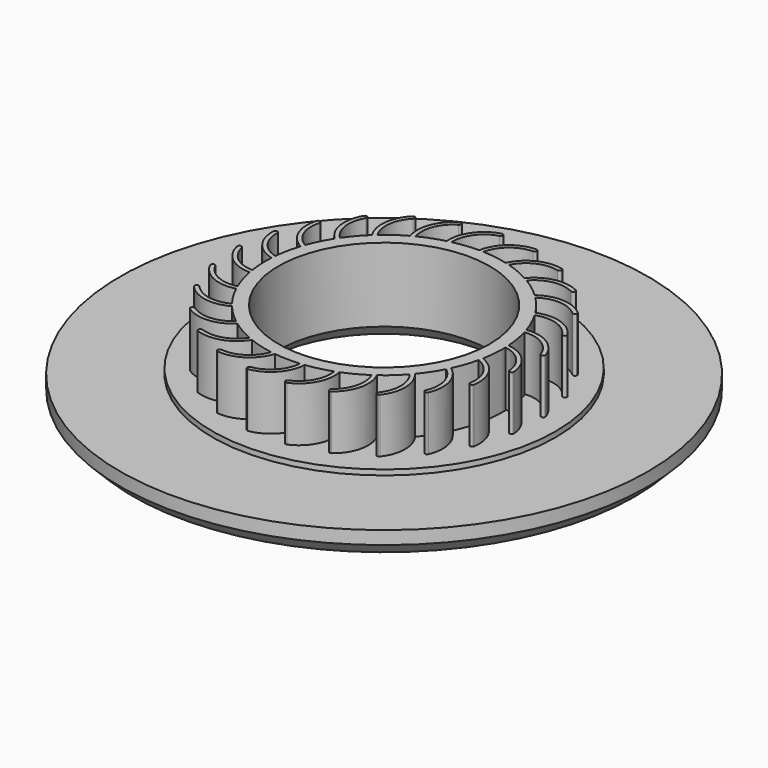
from build123d import *
from build123d import SkipClean  # not in build123d's __all__

# Parameters (mm, degrees)
F0_R     = 50
F1_DEPTH = 5
F2_R     = 32.5
F3_DEPTH = 1
F4_SIZE  = 2.5
F6_DEPTH = 10.5
F7_DEPTH = 0.2
F8_R     = 20
F9_DEPTH = 16.501
F10_SIZE = 2.5


# Not quite as in the source:
# - after a boolean that leaves OpenCascade's solid faulty, fix() repairs it


with BuildPart() as f1:
    # F0 (on Top) → F1 (new body)
    with BuildSketch(Plane.XY):
        Circle(F0_R)
    extrude(amount=F1_DEPTH)

    # F2 (on face) → F3 (join)
    with BuildSketch(Plane.XY.offset(5)):
        Circle(F2_R)
    extrude(amount=F3_DEPTH)

    # F4
    f4_edges = [f1.edges().sort_by_distance(p)[0] for p in [
        (-50, 0, 0),
    ]]
    chamfer(f4_edges, length=F4_SIZE)

    # F5 (on face) → F6 (join)
    with BuildSketch(Plane.XY.offset(6)):
        with BuildLine():
            ThreePointArc((22.4919640181, 0.601294112), (22.4774451189, 1.0072045119), (22.4556013896, 1.4127866894))
            ThreePointArc((22.4556013896, 1.4127866894), (22.1739675521, 3.8164332825), (21.6358018438, 6.1759273455))
            ThreePointArc((21.6358018438, 6.1759273455), (21.5207932709, 6.5654746204), (21.3987716166, 6.9528823734))
            ThreePointArc((21.3987716166, 6.9528823734), (20.528223224, 9.2109745015), (19.4201826687, 11.3625043505))
            ThreePointArc((19.4201826687, 11.3625043505), (19.2119108338, 11.7112118124), (18.9973783238, 12.056102887))
            ThreePointArc((18.9973783238, 12.056102887), (17.5926151331, 14.026756317), (15.9843219941, 15.8351334187))
            ThreePointArc((15.9843219941, 15.8351334187), (15.6958733825, 16.1210904954), (15.4023098834, 16.401794117))
            ThreePointArc((15.4023098834, 16.401794117), (13.5515983324, 17.9611854463), (11.5441075824, 19.3127828167))
            ThreePointArc((11.5441075824, 19.3127828167), (11.1936064813, 19.5180217733), (10.8394576673, 19.716900301))
            ThreePointArc((10.8394576673, 19.716900301), (8.6590847692, 20.7670472374), (6.3785344351, 21.5769390429))
            ThreePointArc((6.3785344351, 21.5769390429), (5.9880041176, 21.6885639609), (5.5955224612, 21.7931211254))
            ThreePointArc((5.5955224612, 21.7931211254), (3.222489064, 22.2680390747), (0.8121745106, 22.4853368346))
            ThreePointArc((0.8121745106, 22.4853368346), (0.4061534328, 22.49633391), (0, 22.5))
            ThreePointArc((0, 22.5), (-2.4165874806, 22.3698481208), (-4.8052173254, 21.9808982177))
            ThreePointArc((-4.8052173254, 21.9808982177), (-5.2012173658, 21.8905764637), (-5.5955224612, 21.7931211254))
            ThreePointArc((-5.5955224612, 21.7931211254), (-7.9038209461, 21.066077339), (-10.1206796845, 20.0953189256))
            ThreePointArc((-10.1206796845, 20.0953189256), (-10.4817765486, 19.9093535903), (-10.8394576673, 19.716900301))
            ThreePointArc((-10.8394576673, 19.716900301), (-12.8944282734, 18.4386474423), (-14.8002225178, 16.9470768401))
            ThreePointArc((-14.8002225178, 16.9470768401), (-15.1037271616, 16.6771528094), (-15.4023098834, 16.401794117))
            ThreePointArc((-15.4023098834, 16.401794117), (-17.0748312499, 14.6526495142), (-18.5498129388, 12.7339875897))
            ThreePointArc((-18.5498129388, 12.7339875897), (-18.7766550494, 12.3970651831), (-18.9973783238, 12.056102887))
            ThreePointArc((-18.9973783238, 12.056102887), (-20.1823597822, 9.9459717285), (-21.1338503915, 7.7207750668))
            ThreePointArc((-21.1338503915, 7.7207750668), (-21.2697766448, 7.3380243582), (-21.3987716166, 6.9528823734))
            ThreePointArc((-21.3987716166, 6.9528823734), (-22.0217564237, 4.6143519603), (-22.3899702992, 2.2224378513))
            ThreePointArc((-22.3899702992, 2.2224378513), (-22.4264399487, 1.8179084755), (-22.4556013896, 1.4127866894))
            ThreePointArc((-22.4556013896, 1.4127866894), (-22.4774451189, -1.0072045119), (-22.2392460284, -3.4155433079))
            ThreePointArc((-22.2392460284, -3.4155433079), (-22.1739675521, -3.8164332825), (-22.1014631414, -4.2160795782))
            ThreePointArc((-22.1014631414, -4.2160795782), (-21.5207932709, -6.5654746204), (-20.6911481395, -8.8389133196))
            ThreePointArc((-20.6911481395, -8.8389133196), (-20.528223224, -9.2109745015), (-20.3586086805, -9.5800340602))
            ThreePointArc((-20.3586086805, -9.5800340602), (-19.2119108338, -11.7112118124), (-17.8429493162, -13.7069019001))
            ThreePointArc((-17.8429493162, -13.7069019001), (-17.5926151331, -14.026756317), (-17.3365479625, -14.3420397693))
            ThreePointArc((-17.3365479625, -14.3420397693), (-15.6958733825, -16.1210904954), (-13.8736123656, -17.7136354238))
            ThreePointArc((-13.8736123656, -17.7136354238), (-13.5515983324, -17.9611854463), (-13.2251681766, -18.2028823734))
            ThreePointArc((-13.2251681766, -18.2028823734), (-11.1936064813, -19.5180217733), (-9.0325453265, -20.6073560877))
            ThreePointArc((-9.0325453265, -20.6073560877), (-8.6590847692, -20.7670472374), (-8.2828024354, -20.9199709325))
            ThreePointArc((-8.2828024354, -20.9199709325), (-5.9880041176, -21.6885639609), (-3.6239302452, -22.20624078))
            ThreePointArc((-3.6239302452, -22.20624078), (-3.222489064, -22.2680390747), (-2.8199977552, -22.3225807796))
            ThreePointArc((-2.8199977552, -22.3225807796), (-0.4061534328, -22.49633391), (2.0123897013, -22.4098256952))
            ThreePointArc((2.0123897013, -22.4098256952), (2.4165874806, -22.3698481208), (2.8199977552, -22.3225807796))
            ThreePointArc((2.8199977552, -22.3225807796), (5.2012173658, -21.8905764637), (7.5222638018, -21.2053188445))
            ThreePointArc((7.5222638018, -21.2053188445), (7.9038209461, -21.066077339), (8.2828024354, -20.9199709325))
            ThreePointArc((8.2828024354, -20.9199709325), (10.4817765486, -19.9093535903), (12.5594864028, -18.668403823))
            ThreePointArc((12.5594864028, -18.668403823), (12.8944282734, -18.4386474423), (13.2251681766, -18.2028823734))
            ThreePointArc((13.2251681766, -18.2028823734), (15.1037271616, -16.6771528094), (16.8075502824, -14.9584843318))
            ThreePointArc((16.8075502824, -14.9584843318), (17.0748312499, -14.6526495142), (17.3365479625, -14.3420397693))
            ThreePointArc((17.3365479625, -14.3420397693), (18.7766550494, -12.3970651831), (19.999533964, -10.3086682565))
            ThreePointArc((19.999533964, -10.3086682565), (20.1823597822, -9.9459717285), (20.3586086805, -9.5800340602))
            ThreePointArc((20.3586086805, -9.5800340602), (21.2697766448, -7.3380243582), (21.9348733735, -5.011120642))
            ThreePointArc((21.9348733735, -5.011120642), (22.0217564237, -4.6143519603), (22.1014631414, -4.2160795782))
            ThreePointArc((22.1014631414, -4.2160795782), (22.4001442036, -2.1174370497), (22.5, 0))
            ThreePointArc((22.5, 0), (22.4979909148, 0.300673904), (22.4919640181, 0.601294112))
        make_face()
        with BuildLine():
            ThreePointArc((-13.9116834444, 24.2717188462), (-13.846454671, 24.7564653989), (-14.2990440405, 24.9419293466))
            ThreePointArc((-14.2990440405, 24.9419293466), (-14.386541076, 24.8915635481), (-14.4738607094, 24.8408908086))
            ThreePointArc((-14.4738607094, 24.8408908086), (-16.4354533618, 20.7860793054), (-15.4023098834, 16.401794117))
            ThreePointArc((-15.4023098834, 16.401794117), (-15.1037271616, 16.6771528094), (-14.8002225178, 16.9470768401))
            ThreePointArc((-14.8002225178, 16.9470768401), (-15.6326549951, 20.7642722553), (-13.9116834444, 24.2717188462))
        make_face()
        with BuildLine():
            ThreePointArc((-7.438491306, 26.9688731522), (-7.254760249, 27.4221687642), (-7.647007683, 27.7143604201))
            ThreePointArc((-7.647007683, 27.7143604201), (-7.744281303, 27.6873365837), (-7.8414594274, 27.6599713313))
            ThreePointArc((-7.8414594274, 27.6599713313), (-10.7498156547, 24.2203774431), (-10.8394576673, 19.716900301))
            ThreePointArc((-10.8394576673, 19.716900301), (-10.4817765486, 19.9093535903), (-10.1206796845, 20.0953189256))
            ThreePointArc((-10.1206796845, 20.0953189256), (-9.9776618678, 23.9996076664), (-7.438491306, 26.9688731522))
        make_face()
        with BuildLine():
            ThreePointArc((-0.4979114021, 27.9714739734), (-0.2072225594, 28.3648364144), (-0.514481709, 28.7453963022))
            ThreePointArc((-0.514481709, 28.7453963022), (-0.6154198542, 28.7434124349), (-0.7163504107, 28.741074129))
            ThreePointArc((-0.7163504107, 28.741074129), (-4.3887274949, 26.1328201898), (-5.5955224612, 21.7931211254))
            ThreePointArc((-5.5955224612, 21.7931211254), (-5.2012173658, 21.8905764637), (-4.8052173254, 21.9808982177))
            ThreePointArc((-4.8052173254, 21.9808982177), (-3.69573555, 25.7269594634), (-0.4979114021, 27.9714739734))
        make_face()
        with BuildLine():
            ThreePointArc((6.4739541065, 27.216524213), (6.8533356857, 27.5252370741), (6.6503710429, 27.9702532165))
            ThreePointArc((6.6503710429, 27.9702532165), (6.5521106873, 27.9934339719), (6.4537695369, 28.0162695369))
            ThreePointArc((6.4537695369, 28.0162695369), (2.2481205539, 26.4032417342), (0, 22.5))
            ThreePointArc((0, 22.5), (0.4061534328, 22.49633391), (0.8121745106, 22.4853368346))
            ThreePointArc((0.8121745106, 22.4853368346), (2.8184074243, 25.8377917802), (6.4739541065, 27.216524213))
        make_face()
        with BuildLine():
            ThreePointArc((13.039037269, 24.7514601409), (13.4832736448, 24.9561258576), (13.3973565237, 25.4376362537))
            ThreePointArc((13.3973565237, 25.4376362537), (13.3079480174, 25.4845250999), (13.2183754092, 25.5310996932))
            ThreePointArc((13.2183754092, 25.5310996932), (8.7437109204, 25.014650496), (5.5955224612, 21.7931211254))
            ThreePointArc((5.5955224612, 21.7931211254), (5.9880041176, 21.6885639609), (6.3785344351, 21.5769390429))
            ThreePointArc((6.3785344351, 21.5769390429), (9.1554594948, 24.3251406147), (13.039037269, 24.7514601409))
        make_face()
        with BuildLine():
            ThreePointArc((18.7848297657, 20.7311707986), (19.2660079329, 20.8189294714), (19.3025368222, 21.3066790521))
            ThreePointArc((19.3025368222, 21.3066790521), (19.2275980304, 21.3743297902), (19.1524221407, 21.4417169589))
            ThreePointArc((19.1524221407, 21.4417169589), (14.6899017726, 22.0542967698), (10.8394576673, 19.716900301))
            ThreePointArc((10.8394576673, 19.716900301), (11.1936064813, 19.5180217733), (11.5441075824, 19.3127828167))
            ThreePointArc((11.5441075824, 19.3127828167), (14.9172403738, 21.2840514028), (18.7848297657, 20.7311707986))
        make_face()
        with BuildLine():
            ThreePointArc((23.3503023224, 15.4082657512), (23.8381880871, 15.3736031798), (23.9948677424, 15.8369448451))
            ThreePointArc((23.9948677424, 15.8369448451), (23.9391073449, 15.9211067306), (23.8830517514, 16.005072291))
            ThreePointArc((23.8830517514, 16.005072291), (19.7130720707, 17.7081904675), (15.4023098834, 16.401794117))
            ThreePointArc((15.4023098834, 16.401794117), (15.6958733825, 16.1210904954), (15.9843219941, 15.8351334187))
            ThreePointArc((15.9843219941, 15.8351334187), (19.7417161784, 16.905606964), (23.3503023224, 15.4082657512))
        make_face()
        with BuildLine():
            ThreePointArc((26.4485895078, 9.117202699), (26.9125272131, 8.9622968602), (27.1795128753, 9.3721171493))
            ThreePointArc((27.1795128753, 9.3721171493), (27.1464345031, 9.4675019813), (27.1130213849, 9.5627700685))
            ThreePointArc((27.1130213849, 9.5627700685), (23.4975975511, 12.2494134319), (18.9973783238, 12.056102887))
            ThreePointArc((18.9973783238, 12.056102887), (19.2119108338, 11.7112118124), (19.4201826687, 11.3625043505))
            ThreePointArc((19.4201826687, 11.3625043505), (23.3257473505, 11.4649210651), (26.4485895078, 9.117202699))
        make_face()
        with BuildLine():
            ThreePointArc((27.8850145434, 2.2532722704), (28.2958532769, 1.9878564679), (28.6563692551, 2.3184048648))
            ThreePointArc((28.6563692551, 2.3184048648), (28.6480513439, 2.4190192636), (28.63938017, 2.5196038332))
            ThreePointArc((28.63938017, 2.5196038332), (25.8056825592, 6.0209607002), (21.3987716166, 6.9528823734))
            ThreePointArc((21.3987716166, 6.9528823734), (21.5207932709, 6.5654746204), (21.6358018438, 6.1759273455))
            ThreePointArc((21.6358018438, 6.1759273455), (25.4441360304, 5.3038520107), (27.8850145434, 2.2532722704))
        make_face()
        with BuildLine():
            ThreePointArc((28.3326405638, -4.8809813239), (28.3496057586, -4.7814593311), (28.3662213708, -4.6818783775))
            ThreePointArc((28.3662213708, -4.6818783775), (26.4923016254, -0.5858111358), (22.4556013896, 1.4127866894))
            ThreePointArc((22.4556013896, 1.4127866894), (22.4774451189, 1.0072045119), (22.4919640181, 0.601294112))
            ThreePointArc((22.4919640181, 0.601294112), (25.9637760666, -1.1904775717), (27.5693215612, -4.7522395418))
            ThreePointArc((27.5693215612, -4.7522395418), (27.9012468145, -5.1114882571), (28.3326405638, -4.8809813239))
        make_face()
        with BuildLine():
            ThreePointArc((26.2286678657, -11.773677505), (26.2698501808, -11.681501251), (26.3107085592, -11.5891809509))
            ThreePointArc((26.3107085592, -11.5891809509), (25.5143119486, -7.1557743037), (22.1014631414, -4.2160795782))
            ThreePointArc((22.1014631414, -4.2160795782), (22.0217564237, -4.6143519603), (21.9348733735, -5.011120642))
            ThreePointArc((21.9348733735, -5.011120642), (24.8520165645, -7.61000507), (25.5213467125, -11.4591506661))
            ThreePointArc((25.5213467125, -11.4591506661), (25.7535024011, -11.8896593762), (26.2286678657, -11.773677505))
        make_face()
        with BuildLine():
            ThreePointArc((22.4766515033, -17.9265902279), (22.5394633025, -17.8475514857), (22.6019971648, -17.7682926631))
            ThreePointArc((22.6019971648, -17.7682926631), (22.9331642171, -13.276113855), (20.3586086805, -9.5800340602))
            ThreePointArc((20.3586086805, -9.5800340602), (20.1823597822, -9.9459717285), (19.999533964, -10.3086682565))
            ThreePointArc((19.999533964, -10.3086682565), (22.1787134623, -13.5513679622), (21.8697717889, -17.4460412103))
            ThreePointArc((21.8697717889, -17.4460412103), (21.9875707171, -17.9207594696), (22.4766515033, -17.9265902279))
        make_face()
        with BuildLine():
            ThreePointArc((17.3123444636, -22.9531093574), (17.3928390506, -22.8921744219), (17.4731191642, -22.8309572001))
            ThreePointArc((17.4731191642, -22.8309572001), (18.9110414355, -18.5622663467), (17.3365479625, -14.3420397693))
            ThreePointArc((17.3365479625, -14.3420397693), (17.0748312499, -14.6526495142), (16.8075502824, -14.9584843318))
            ThreePointArc((16.8075502824, -14.9584843318), (18.1118402256, -18.6412485668), (16.8440386724, -22.3367328231))
            ThreePointArc((16.8440386724, -22.3367328231), (16.8400791003, -22.8258323375), (17.3123444636, -22.9531093574))
        make_face()
        with BuildLine():
            ThreePointArc((11.0602391509, -26.5374002103), (11.1533587547, -26.4983978476), (11.2463408249, -26.4590687298))
            ThreePointArc((11.2463408249, -26.4590687298), (13.7006683705, -22.6820833765), (13.2251681766, -18.2028823734))
            ThreePointArc((13.2251681766, -18.2028823734), (12.8944282734, -18.4386474423), (12.5594864028, -18.668403823))
            ThreePointArc((12.5594864028, -18.668403823), (12.9069334569, -22.5598309663), (10.7599326581, -25.8239253639))
            ThreePointArc((10.7599326581, -25.8239253639), (10.6344633801, -26.2966742122), (11.0602391509, -26.5374002103))
        make_face()
        with BuildLine():
            ThreePointArc((4.1131783357, -28.4542486103), (4.213071909, -28.4396294823), (4.3129135304, -28.4246596616))
            ThreePointArc((4.3129135304, -28.4246596616), (7.6294319243, -25.376701689), (8.2828024354, -20.9199709325))
            ThreePointArc((8.2828024354, -20.9199709325), (7.9038209461, -21.066077339), (7.5222638018, -21.2053188445))
            ThreePointArc((7.5222638018, -21.2053188445), (6.8910365907, -25.0608962169), (3.9997405026, -27.6885057004))
            ThreePointArc((3.9997405026, -27.6885057004), (3.760645215, -28.1151993337), (4.1131783357, -28.4542486103))
        make_face()
        with BuildLine():
            ThreePointArc((-3.0923286016, -28.5832119227), (-2.9919377393, -28.5938946029), (-2.891509983, -28.6042246883))
            ThreePointArc((-2.891509983, -28.6042246883), (1.0788102112, -26.4768085053), (2.8199977552, -22.3225807796))
            ThreePointArc((2.8199977552, -22.3225807796), (2.4165874806, -22.3698481208), (2.0123897013, -22.4098256952))
            ThreePointArc((2.0123897013, -22.4098256952), (0.442150552, -25.9872931907), (-3.0117700587, -27.8133153925))
            ThreePointArc((-3.0117700587, -27.8133153925), (-3.3494681197, -28.1671430805), (-3.0923286016, -28.5832119227))
        make_face()
        with BuildLine():
            ThreePointArc((-10.10353316, -26.9161869083), (-10.0089529358, -26.9515001647), (-9.9142492899, -26.9864810788))
            ThreePointArc((-9.9142492899, -26.9864810788), (-5.539597115, -25.9132800684), (-2.8199977552, -22.3225807796))
            ThreePointArc((-2.8199977552, -22.3225807796), (-3.222489064, -22.2680390747), (-3.6239302452, -22.20624078))
            ThreePointArc((-3.6239302452, -22.20624078), (-6.0345174319, -25.2808129587), (-9.8340400307, -26.1905121883))
            ThreePointArc((-9.8340400307, -26.1905121883), (-10.2491220539, -26.4492416362), (-10.10353316, -26.9161869083))
        make_face()
        with BuildLine():
            ThreePointArc((-16.4798955719, -23.5579188797), (-16.397068809, -23.6156438505), (-16.3140398519, -23.6730776138))
            ThreePointArc((-16.3140398519, -23.6730776138), (-11.8099311813, -23.7215249424), (-8.2828024354, -20.9199709325))
            ThreePointArc((-8.2828024354, -20.9199709325), (-8.6590847692, -20.7670472374), (-9.0325453265, -20.6073560877))
            ThreePointArc((-9.0325453265, -20.6073560877), (-12.1320144922, -22.9858462722), (-16.0384011005, -22.9220627813))
            ThreePointArc((-16.0384011005, -22.9220627813), (-16.5047859559, -23.0694370663), (-16.4798955719, -23.5579188797))
        make_face()
        with BuildLine():
            ThreePointArc((-21.8207655361, -18.7194201678), (-21.7548965448, -18.7959297808), (-21.6887592912, -18.8722076189))
            ThreePointArc((-21.6887592912, -18.8722076189), (-17.3382038376, -20.0392591626), (-13.2251681766, -18.2028823734))
            ThreePointArc((-13.2251681766, -18.2028823734), (-13.5515983324, -17.9611854463), (-13.8736123656, -17.7136354238))
            ThreePointArc((-13.8736123656, -17.7136354238), (-17.4672124636, -19.2465943284), (-21.235010444, -18.2133358683))
            ThreePointArc((-21.235010444, -18.2133358683), (-21.7233934559, -18.2400949221), (-21.8207655361, -18.7194201678))
        make_face()
        with BuildLine():
            ThreePointArc((-25.7905565505, -12.7047114416), (-25.7457841217, -12.7951983164), (-25.7006942185, -12.8855274121))
            ThreePointArc((-25.7006942185, -12.8855274121), (-21.7770533813, -15.0978530303), (-17.3365479625, -14.3420397693))
            ThreePointArc((-17.3365479625, -14.3420397693), (-17.5926151331, -14.026756317), (-17.8429493162, -13.7069019001))
            ThreePointArc((-17.8429493162, -13.7069019001), (-21.7048812359, -14.2980080789), (-25.0973459844, -12.3601980787))
            ThreePointArc((-25.0973459844, -12.3601980787), (-25.577040252, -12.2646605315), (-25.7905565505, -12.7047114416))
        make_face()
        with BuildLine():
            ThreePointArc((-28.1398320458, -5.8917189709), (-28.1189693959, -5.9904974844), (-28.0977600075, -6.0892021283))
            ThreePointArc((-28.0977600075, -6.0892021283), (-24.8475705707, -9.2077932662), (-20.3586086805, -9.5800340602))
            ThreePointArc((-20.3586086805, -9.5800340602), (-20.528223224, -9.2109745015), (-20.6911481395, -8.8389133196))
            ThreePointArc((-20.6911481395, -8.8389133196), (-24.5787524952, -8.4510253974), (-27.3827229751, -5.7304235863))
            ThreePointArc((-27.3827229751, -5.7304235863), (-27.8235875433, -5.5185924135), (-28.1398320458, -5.8917189709))
        make_face()
        with BuildLine():
            ThreePointArc((-28.7209784027, 1.291471871), (-28.7253364086, 1.1906083361), (-28.7293401989, 1.0897301196))
            ThreePointArc((-28.7293401989, 1.0897301196), (-26.3568235181, -2.7391739872), (-22.1014631414, -4.2160795782))
            ThreePointArc((-22.1014631414, -4.2160795782), (-22.1739675521, -3.8164332825), (-22.2392460284, -3.4155433079))
            ThreePointArc((-22.2392460284, -3.4155433079), (-25.9082503409, -2.0730337095), (-27.9475427746, 1.2594144951))
            ThreePointArc((-27.9475427746, 1.2594144951), (-28.3218765012, 1.5742291618), (-28.7209784027, 1.291471871))
        make_face()
        with BuildLine():
            ThreePointArc((-26.7563156777, 8.170118932), (-27.040597798, 8.5681361292), (-27.4974800581, 8.3935147856))
            ThreePointArc((-27.4974800581, 8.3935147856), (-27.5267848904, 8.2969038561), (-27.5557502865, 8.2001906164))
            ThreePointArc((-27.5557502865, 8.2001906164), (-26.2099803103, 3.9015576673), (-22.4556013896, 1.4127866894))
            ThreePointArc((-22.4556013896, 1.4127866894), (-22.4264399487, 1.8179084755), (-22.3899702992, 2.2224378513))
            ThreePointArc((-22.3899702992, 2.2224378513), (-25.6098375338, 4.4352143104), (-26.7563156777, 8.170118932))
        make_face()
        with BuildLine():
            ThreePointArc((-23.8838908639, 14.5674647488), (-24.0602588868, 15.0236755923), (-24.5462139128, 14.9681622969))
            ThreePointArc((-24.5462139128, 14.9681622969), (-24.5986242411, 14.8818743929), (-24.6507312407, 14.7954029786))
            ThreePointArc((-24.6507312407, 14.7954029786), (-24.416267646, 10.2971401047), (-21.3987716166, 6.9528823734))
            ThreePointArc((-21.3987716166, 6.9528823734), (-21.2697766448, 7.3380243582), (-21.1338503915, 7.7207750668))
            ThreePointArc((-21.1338503915, 7.7207750668), (-23.7022644481, 10.6647815037), (-23.8838908639, 14.5674647488))
        make_face()
        with BuildLine():
            ThreePointArc((-19.5107533484, 20.0494831801), (-19.5681254223, 20.5352222647), (-20.0526188727, 20.6023051222))
            ThreePointArc((-20.0526188727, 20.6023051222), (-20.1248415633, 20.5317620299), (-20.1968160919, 20.460965758))
            ThreePointArc((-20.1968160919, 20.460965758), (-21.0883910888, 16.0457153591), (-18.9973783238, 12.056102887))
            ThreePointArc((-18.9973783238, 12.056102887), (-18.7766550494, 12.3970651831), (-18.5498129388, 12.7339875897))
            ThreePointArc((-18.5498129388, 12.7339875897), (-20.3053909162, 16.2242412527), (-19.5107533484, 20.0494831801))
        make_face()
    extrude(amount=F6_DEPTH)

    # F5 (on face) → F7 (cut)
    with BuildSketch(Plane.XY.offset(6)):
        with BuildLine():
            ThreePointArc((-10.10353316, -26.9161869083), (-10.0089529358, -26.9515001647), (-9.9142492899, -26.9864810788))
            ThreePointArc((-9.9142492899, -26.9864810788), (-5.539597115, -25.9132800684), (-2.8199977552, -22.3225807796))
            ThreePointArc((-2.8199977552, -22.3225807796), (-3.222489064, -22.2680390747), (-3.6239302452, -22.20624078))
            ThreePointArc((-3.6239302452, -22.20624078), (-6.0345174319, -25.2808129587), (-9.8340400307, -26.1905121883))
            ThreePointArc((-9.8340400307, -26.1905121883), (-10.2491220539, -26.4492416362), (-10.10353316, -26.9161869083))
        make_face()
        with BuildLine():
            ThreePointArc((-16.4798955719, -23.5579188797), (-16.397068809, -23.6156438505), (-16.3140398519, -23.6730776138))
            ThreePointArc((-16.3140398519, -23.6730776138), (-11.8099311813, -23.7215249424), (-8.2828024354, -20.9199709325))
            ThreePointArc((-8.2828024354, -20.9199709325), (-8.6590847692, -20.7670472374), (-9.0325453265, -20.6073560877))
            ThreePointArc((-9.0325453265, -20.6073560877), (-12.1320144922, -22.9858462722), (-16.0384011005, -22.9220627813))
            ThreePointArc((-16.0384011005, -22.9220627813), (-16.5047859559, -23.0694370663), (-16.4798955719, -23.5579188797))
        make_face()
        with BuildLine():
            ThreePointArc((-21.8207655361, -18.7194201678), (-21.7548965448, -18.7959297808), (-21.6887592912, -18.8722076189))
            ThreePointArc((-21.6887592912, -18.8722076189), (-17.3382038376, -20.0392591626), (-13.2251681766, -18.2028823734))
            ThreePointArc((-13.2251681766, -18.2028823734), (-13.5515983324, -17.9611854463), (-13.8736123656, -17.7136354238))
            ThreePointArc((-13.8736123656, -17.7136354238), (-17.4672124636, -19.2465943284), (-21.235010444, -18.2133358683))
            ThreePointArc((-21.235010444, -18.2133358683), (-21.7233934559, -18.2400949221), (-21.8207655361, -18.7194201678))
        make_face()
        with BuildLine():
            ThreePointArc((-25.7905565505, -12.7047114416), (-25.7457841217, -12.7951983164), (-25.7006942185, -12.8855274121))
            ThreePointArc((-25.7006942185, -12.8855274121), (-21.7770533813, -15.0978530303), (-17.3365479625, -14.3420397693))
            ThreePointArc((-17.3365479625, -14.3420397693), (-17.5926151331, -14.026756317), (-17.8429493162, -13.7069019001))
            ThreePointArc((-17.8429493162, -13.7069019001), (-21.7048812359, -14.2980080789), (-25.0973459844, -12.3601980787))
            ThreePointArc((-25.0973459844, -12.3601980787), (-25.577040252, -12.2646605315), (-25.7905565505, -12.7047114416))
        make_face()
        with BuildLine():
            ThreePointArc((-28.1398320458, -5.8917189709), (-28.1189693959, -5.9904974844), (-28.0977600075, -6.0892021283))
            ThreePointArc((-28.0977600075, -6.0892021283), (-24.8475705707, -9.2077932662), (-20.3586086805, -9.5800340602))
            ThreePointArc((-20.3586086805, -9.5800340602), (-20.528223224, -9.2109745015), (-20.6911481395, -8.8389133196))
            ThreePointArc((-20.6911481395, -8.8389133196), (-24.5787524952, -8.4510253974), (-27.3827229751, -5.7304235863))
            ThreePointArc((-27.3827229751, -5.7304235863), (-27.8235875433, -5.5185924135), (-28.1398320458, -5.8917189709))
        make_face()
        with BuildLine():
            ThreePointArc((-28.7209784027, 1.291471871), (-28.7253364086, 1.1906083361), (-28.7293401989, 1.0897301196))
            ThreePointArc((-28.7293401989, 1.0897301196), (-26.3568235181, -2.7391739872), (-22.1014631414, -4.2160795782))
            ThreePointArc((-22.1014631414, -4.2160795782), (-22.1739675521, -3.8164332825), (-22.2392460284, -3.4155433079))
            ThreePointArc((-22.2392460284, -3.4155433079), (-25.9082503409, -2.0730337095), (-27.9475427746, 1.2594144951))
            ThreePointArc((-27.9475427746, 1.2594144951), (-28.3218765012, 1.5742291618), (-28.7209784027, 1.291471871))
        make_face()
        with BuildLine():
            ThreePointArc((-26.7563156777, 8.170118932), (-27.040597798, 8.5681361292), (-27.4974800581, 8.3935147856))
            ThreePointArc((-27.4974800581, 8.3935147856), (-27.5267848904, 8.2969038561), (-27.5557502865, 8.2001906164))
            ThreePointArc((-27.5557502865, 8.2001906164), (-26.2099803103, 3.9015576673), (-22.4556013896, 1.4127866894))
            ThreePointArc((-22.4556013896, 1.4127866894), (-22.4264399487, 1.8179084755), (-22.3899702992, 2.2224378513))
            ThreePointArc((-22.3899702992, 2.2224378513), (-25.6098375338, 4.4352143104), (-26.7563156777, 8.170118932))
        make_face()
        with BuildLine():
            ThreePointArc((-23.8838908639, 14.5674647488), (-24.0602588868, 15.0236755923), (-24.5462139128, 14.9681622969))
            ThreePointArc((-24.5462139128, 14.9681622969), (-24.5986242411, 14.8818743929), (-24.6507312407, 14.7954029786))
            ThreePointArc((-24.6507312407, 14.7954029786), (-24.416267646, 10.2971401047), (-21.3987716166, 6.9528823734))
            ThreePointArc((-21.3987716166, 6.9528823734), (-21.2697766448, 7.3380243582), (-21.1338503915, 7.7207750668))
            ThreePointArc((-21.1338503915, 7.7207750668), (-23.7022644481, 10.6647815037), (-23.8838908639, 14.5674647488))
        make_face()
        with BuildLine():
            ThreePointArc((-19.5107533484, 20.0494831801), (-19.5681254223, 20.5352222647), (-20.0526188727, 20.6023051222))
            ThreePointArc((-20.0526188727, 20.6023051222), (-20.1248415633, 20.5317620299), (-20.1968160919, 20.460965758))
            ThreePointArc((-20.1968160919, 20.460965758), (-21.0883910888, 16.0457153591), (-18.9973783238, 12.056102887))
            ThreePointArc((-18.9973783238, 12.056102887), (-18.7766550494, 12.3970651831), (-18.5498129388, 12.7339875897))
            ThreePointArc((-18.5498129388, 12.7339875897), (-20.3053909162, 16.2242412527), (-19.5107533484, 20.0494831801))
        make_face()
        with BuildLine():
            ThreePointArc((-13.9116834444, 24.2717188462), (-13.846454671, 24.7564653989), (-14.2990440405, 24.9419293466))
            ThreePointArc((-14.2990440405, 24.9419293466), (-14.386541076, 24.8915635481), (-14.4738607094, 24.8408908086))
            ThreePointArc((-14.4738607094, 24.8408908086), (-16.4354533618, 20.7860793054), (-15.4023098834, 16.401794117))
            ThreePointArc((-15.4023098834, 16.401794117), (-15.1037271616, 16.6771528094), (-14.8002225178, 16.9470768401))
            ThreePointArc((-14.8002225178, 16.9470768401), (-15.6326549951, 20.7642722553), (-13.9116834444, 24.2717188462))
        make_face()
        with BuildLine():
            ThreePointArc((-7.438491306, 26.9688731522), (-7.254760249, 27.4221687642), (-7.647007683, 27.7143604201))
            ThreePointArc((-7.647007683, 27.7143604201), (-7.744281303, 27.6873365837), (-7.8414594274, 27.6599713313))
            ThreePointArc((-7.8414594274, 27.6599713313), (-10.7498156547, 24.2203774431), (-10.8394576673, 19.716900301))
            ThreePointArc((-10.8394576673, 19.716900301), (-10.4817765486, 19.9093535903), (-10.1206796845, 20.0953189256))
            ThreePointArc((-10.1206796845, 20.0953189256), (-9.9776618678, 23.9996076664), (-7.438491306, 26.9688731522))
        make_face()
        with BuildLine():
            ThreePointArc((-0.4979114021, 27.9714739734), (-0.2072225594, 28.3648364144), (-0.514481709, 28.7453963022))
            ThreePointArc((-0.514481709, 28.7453963022), (-0.6154198542, 28.7434124349), (-0.7163504107, 28.741074129))
            ThreePointArc((-0.7163504107, 28.741074129), (-4.3887274949, 26.1328201898), (-5.5955224612, 21.7931211254))
            ThreePointArc((-5.5955224612, 21.7931211254), (-5.2012173658, 21.8905764637), (-4.8052173254, 21.9808982177))
            ThreePointArc((-4.8052173254, 21.9808982177), (-3.69573555, 25.7269594634), (-0.4979114021, 27.9714739734))
        make_face()
        with BuildLine():
            ThreePointArc((6.4739541065, 27.216524213), (6.8533356857, 27.5252370741), (6.6503710429, 27.9702532165))
            ThreePointArc((6.6503710429, 27.9702532165), (6.5521106873, 27.9934339719), (6.4537695369, 28.0162695369))
            ThreePointArc((6.4537695369, 28.0162695369), (2.2481205539, 26.4032417342), (0, 22.5))
            ThreePointArc((0, 22.5), (0.4061534328, 22.49633391), (0.8121745106, 22.4853368346))
            ThreePointArc((0.8121745106, 22.4853368346), (2.8184074243, 25.8377917802), (6.4739541065, 27.216524213))
        make_face()
        with BuildLine():
            ThreePointArc((13.039037269, 24.7514601409), (13.4832736448, 24.9561258576), (13.3973565237, 25.4376362537))
            ThreePointArc((13.3973565237, 25.4376362537), (13.3079480174, 25.4845250999), (13.2183754092, 25.5310996932))
            ThreePointArc((13.2183754092, 25.5310996932), (8.7437109204, 25.014650496), (5.5955224612, 21.7931211254))
            ThreePointArc((5.5955224612, 21.7931211254), (5.9880041176, 21.6885639609), (6.3785344351, 21.5769390429))
            ThreePointArc((6.3785344351, 21.5769390429), (9.1554594948, 24.3251406147), (13.039037269, 24.7514601409))
        make_face()
        with BuildLine():
            ThreePointArc((18.7848297657, 20.7311707986), (19.2660079329, 20.8189294714), (19.3025368222, 21.3066790521))
            ThreePointArc((19.3025368222, 21.3066790521), (19.2275980304, 21.3743297902), (19.1524221407, 21.4417169589))
            ThreePointArc((19.1524221407, 21.4417169589), (14.6899017726, 22.0542967698), (10.8394576673, 19.716900301))
            ThreePointArc((10.8394576673, 19.716900301), (11.1936064813, 19.5180217733), (11.5441075824, 19.3127828167))
            ThreePointArc((11.5441075824, 19.3127828167), (14.9172403738, 21.2840514028), (18.7848297657, 20.7311707986))
        make_face()
        with BuildLine():
            ThreePointArc((23.3503023224, 15.4082657512), (23.8381880871, 15.3736031798), (23.9948677424, 15.8369448451))
            ThreePointArc((23.9948677424, 15.8369448451), (23.9391073449, 15.9211067306), (23.8830517514, 16.005072291))
            ThreePointArc((23.8830517514, 16.005072291), (19.7130720707, 17.7081904675), (15.4023098834, 16.401794117))
            ThreePointArc((15.4023098834, 16.401794117), (15.6958733825, 16.1210904954), (15.9843219941, 15.8351334187))
            ThreePointArc((15.9843219941, 15.8351334187), (19.7417161784, 16.905606964), (23.3503023224, 15.4082657512))
        make_face()
        with BuildLine():
            ThreePointArc((26.4485895078, 9.117202699), (26.9125272131, 8.9622968602), (27.1795128753, 9.3721171493))
            ThreePointArc((27.1795128753, 9.3721171493), (27.1464345031, 9.4675019813), (27.1130213849, 9.5627700685))
            ThreePointArc((27.1130213849, 9.5627700685), (23.4975975511, 12.2494134319), (18.9973783238, 12.056102887))
            ThreePointArc((18.9973783238, 12.056102887), (19.2119108338, 11.7112118124), (19.4201826687, 11.3625043505))
            ThreePointArc((19.4201826687, 11.3625043505), (23.3257473505, 11.4649210651), (26.4485895078, 9.117202699))
        make_face()
        with BuildLine():
            ThreePointArc((27.8850145434, 2.2532722704), (28.2958532769, 1.9878564679), (28.6563692551, 2.3184048648))
            ThreePointArc((28.6563692551, 2.3184048648), (28.6480513439, 2.4190192636), (28.63938017, 2.5196038332))
            ThreePointArc((28.63938017, 2.5196038332), (25.8056825592, 6.0209607002), (21.3987716166, 6.9528823734))
            ThreePointArc((21.3987716166, 6.9528823734), (21.5207932709, 6.5654746204), (21.6358018438, 6.1759273455))
            ThreePointArc((21.6358018438, 6.1759273455), (25.4441360304, 5.3038520107), (27.8850145434, 2.2532722704))
        make_face()
        with BuildLine():
            ThreePointArc((28.3326405638, -4.8809813239), (28.3496057586, -4.7814593311), (28.3662213708, -4.6818783775))
            ThreePointArc((28.3662213708, -4.6818783775), (26.4923016254, -0.5858111358), (22.4556013896, 1.4127866894))
            ThreePointArc((22.4556013896, 1.4127866894), (22.4774451189, 1.0072045119), (22.4919640181, 0.601294112))
            ThreePointArc((22.4919640181, 0.601294112), (25.9637760666, -1.1904775717), (27.5693215612, -4.7522395418))
            ThreePointArc((27.5693215612, -4.7522395418), (27.9012468145, -5.1114882571), (28.3326405638, -4.8809813239))
        make_face()
        with BuildLine():
            ThreePointArc((26.2286678657, -11.773677505), (26.2698501808, -11.681501251), (26.3107085592, -11.5891809509))
            ThreePointArc((26.3107085592, -11.5891809509), (25.5143119486, -7.1557743037), (22.1014631414, -4.2160795782))
            ThreePointArc((22.1014631414, -4.2160795782), (22.0217564237, -4.6143519603), (21.9348733735, -5.011120642))
            ThreePointArc((21.9348733735, -5.011120642), (24.8520165645, -7.61000507), (25.5213467125, -11.4591506661))
            ThreePointArc((25.5213467125, -11.4591506661), (25.7535024011, -11.8896593762), (26.2286678657, -11.773677505))
        make_face()
        with BuildLine():
            ThreePointArc((22.4766515033, -17.9265902279), (22.5394633025, -17.8475514857), (22.6019971648, -17.7682926631))
            ThreePointArc((22.6019971648, -17.7682926631), (22.9331642171, -13.276113855), (20.3586086805, -9.5800340602))
            ThreePointArc((20.3586086805, -9.5800340602), (20.1823597822, -9.9459717285), (19.999533964, -10.3086682565))
            ThreePointArc((19.999533964, -10.3086682565), (22.1787134623, -13.5513679622), (21.8697717889, -17.4460412103))
            ThreePointArc((21.8697717889, -17.4460412103), (21.9875707171, -17.9207594696), (22.4766515033, -17.9265902279))
        make_face()
        with BuildLine():
            ThreePointArc((17.3123444636, -22.9531093574), (17.3928390506, -22.8921744219), (17.4731191642, -22.8309572001))
            ThreePointArc((17.4731191642, -22.8309572001), (18.9110414355, -18.5622663467), (17.3365479625, -14.3420397693))
            ThreePointArc((17.3365479625, -14.3420397693), (17.0748312499, -14.6526495142), (16.8075502824, -14.9584843318))
            ThreePointArc((16.8075502824, -14.9584843318), (18.1118402256, -18.6412485668), (16.8440386724, -22.3367328231))
            ThreePointArc((16.8440386724, -22.3367328231), (16.8400791003, -22.8258323375), (17.3123444636, -22.9531093574))
        make_face()
        with BuildLine():
            ThreePointArc((11.0602391509, -26.5374002103), (11.1533587547, -26.4983978476), (11.2463408249, -26.4590687298))
            ThreePointArc((11.2463408249, -26.4590687298), (13.7006683705, -22.6820833765), (13.2251681766, -18.2028823734))
            ThreePointArc((13.2251681766, -18.2028823734), (12.8944282734, -18.4386474423), (12.5594864028, -18.668403823))
            ThreePointArc((12.5594864028, -18.668403823), (12.9069334569, -22.5598309663), (10.7599326581, -25.8239253639))
            ThreePointArc((10.7599326581, -25.8239253639), (10.6344633801, -26.2966742122), (11.0602391509, -26.5374002103))
        make_face()
        with BuildLine():
            ThreePointArc((4.1131783357, -28.4542486103), (4.213071909, -28.4396294823), (4.3129135304, -28.4246596616))
            ThreePointArc((4.3129135304, -28.4246596616), (7.6294319243, -25.376701689), (8.2828024354, -20.9199709325))
            ThreePointArc((8.2828024354, -20.9199709325), (7.9038209461, -21.066077339), (7.5222638018, -21.2053188445))
            ThreePointArc((7.5222638018, -21.2053188445), (6.8910365907, -25.0608962169), (3.9997405026, -27.6885057004))
            ThreePointArc((3.9997405026, -27.6885057004), (3.760645215, -28.1151993337), (4.1131783357, -28.4542486103))
        make_face()
        with BuildLine():
            ThreePointArc((-3.0923286016, -28.5832119227), (-2.9919377393, -28.5938946029), (-2.891509983, -28.6042246883))
            ThreePointArc((-2.891509983, -28.6042246883), (1.0788102112, -26.4768085053), (2.8199977552, -22.3225807796))
            ThreePointArc((2.8199977552, -22.3225807796), (2.4165874806, -22.3698481208), (2.0123897013, -22.4098256952))
            ThreePointArc((2.0123897013, -22.4098256952), (0.442150552, -25.9872931907), (-3.0117700587, -27.8133153925))
            ThreePointArc((-3.0117700587, -27.8133153925), (-3.3494681197, -28.1671430805), (-3.0923286016, -28.5832119227))
        make_face()
    with SkipClean():  # cleaning this boolean's faces spoils the solid; the shape is the same uncleaned
        extrude(amount=F7_DEPTH, mode=Mode.SUBTRACT)

    # F8 (on face) → F9 (cut, through all)
    with BuildSketch(Plane.XY.offset(16.5)):
        Circle(F8_R)
    extrude(amount=-F9_DEPTH, mode=Mode.SUBTRACT)

    add(f1.part.fix(), mode=Mode.REPLACE)

    # F10
    f10_edges = [f1.edges().sort_by_distance(p)[0] for p in [
        (-20, 0, 0),
    ]]
    chamfer(f10_edges, length=F10_SIZE)


solid = f1.part
